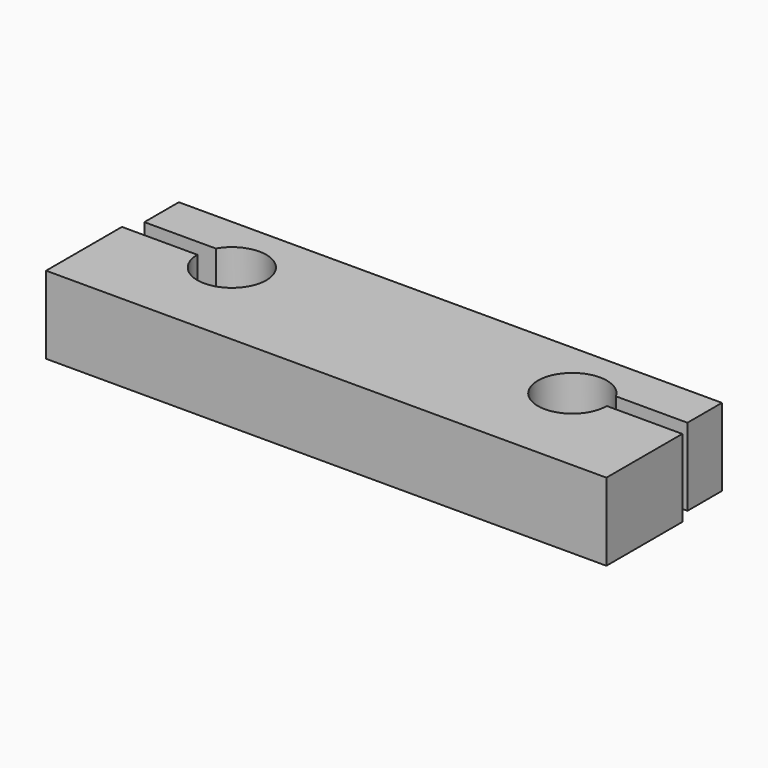
from build123d import *

# Parameters (mm, degrees)
F0_R     = 13
F1_DEPTH = 18
F2_DEPTH = 2
F3_DEPTH = 2


with BuildPart() as f1:
    # F0 (on Top) → F1 (new body)
    with BuildSketch(Plane.XY):
        with BuildLine():
            Line((43.6501808017, 30.4717739075), (-86.3498191983, 30.4717739075))
            Line((-86.3498191983, 30.4717739075), (-86.3498191983, 20.4717739075))
            Line((-86.3498191983, 20.4717739075), (-67.7780224285, 20.4717739075))
            ThreePointArc((-67.7780224285, 20.4717739075), (-58.7792668374, 24.1991805179), (-52.8498191983, 16.4717739075))
            ThreePointArc((-52.8498191983, 16.4717739075), (-60.8498191983, 8.4717739075), (-68.8498191983, 16.4717739075))
            Line((-68.8498191983, 16.4717739075), (-86.3498191983, 16.4717739075))
            Line((-86.3498191983, 16.4717739075), (-86.3498191983, -5.5282260925))
            Line((-86.3498191983, -5.5282260925), (43.6501808017, -5.5282260925))
            Line((43.6501808017, -5.5282260925), (43.6501808017, 16.4717739075))
            Line((43.6501808017, 16.4717739075), (26.1501808017, 16.4717739075))
            ThreePointArc((26.1501808017, 16.4717739075), (10.4227741914, 14.4012215467), (25.078384032, 20.4717739075))
            Line((25.078384032, 20.4717739075), (43.6501808017, 20.4717739075))
            Line((43.6501808017, 20.4717739075), (43.6501808017, 30.4717739075))
        make_face()
        with Locations((-21.3498191983, 16.4717739075)):
            Circle(F0_R, mode=Mode.SUBTRACT)
        with Locations((-21.3498191983, 16.4717739075)):
            Circle(F0_R)
    extrude(amount=F1_DEPTH)

    # F2 (cut): a face of the model
    f2_faces = [f1.faces().sort_by_distance(p)[0] for p in [
        (-86.3498191983, 25.4717739075, 9),
    ]]
    extrude(f2_faces, amount=-F2_DEPTH, mode=Mode.SUBTRACT)

    # F3 (cut): a face of the model
    f3_faces = [f1.faces().sort_by_distance(p)[0] for p in [
        (43.6501808017, 25.4717739075, 9),
    ]]
    extrude(f3_faces, amount=-F3_DEPTH, mode=Mode.SUBTRACT)


solid = f1.part
